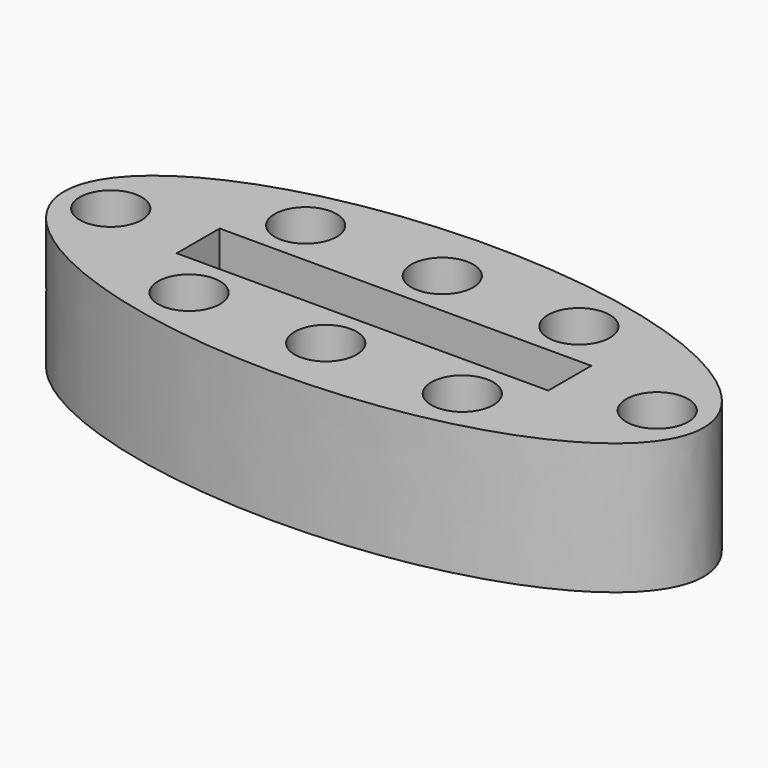
from build123d import *

# Parameters (mm, degrees)
F1_DEPTH = 7.2
F2_W     = 20.4
F2_H     = 2.95
F3_DEPTH = 5.85
F4_W     = 19.15
F4_H     = 1.8
F5_DEPTH = 1.3510001
F6_R     = 1.7
F7_DEPTH = 6.3


# Not quite as in the source:
# - a feature names something its author has since deleted; it is built from what else it names


with BuildPart() as f1:
    # F0 (on Top) → F1 (new body)
    with BuildSketch(Plane.XY):
        with BuildLine():
            add(Edge.make_bspline(
                [(17.5563361044, 0), (17.5563361044, 12.9811752067), (-8.7781680522, 6.4905876034), (-35.1126722087, 0), (-8.7781680522, -6.4905876034), (17.5563361044, -12.9811752067), (17.5563361044, 0)],
                knots=[0, 0, 0, 2.0943951024, 2.0943951024, 4.1887902048, 4.1887902048, 6.2831853072, 6.2831853072, 6.2831853072], degree=2, weights=[1, 0.5, 1, 0.5, 1, 0.5, 1]))
        make_face()
    extrude(amount=F1_DEPTH)

    # F2 (on face) → F3 (cut)
    with BuildSketch(Plane.XY.offset(7.2)):
        Rectangle(F2_W, F2_H)
    extrude(amount=-F3_DEPTH, mode=Mode.SUBTRACT)

    # F4 (on face) → F5 (cut, through all)
    with BuildSketch(Plane.XY.offset(1.35)):
        Rectangle(F4_W, F4_H)
    extrude(amount=-F5_DEPTH, mode=Mode.SUBTRACT)

    # F6 (on face) → F7 (cut)
    with BuildSketch(Plane.XY.offset(7.2)):
        with Locations((-15, 0)):
            Circle(F6_R)
        with Locations((0, 4)):
            Circle(F6_R)
        with Locations((0, -4)):
            Circle(F6_R)
        with Locations((15, 0)):
            Circle(F6_R)
        with Locations((-7.5, 4)):
            Circle(F6_R)
        with Locations((7.5, 4)):
            Circle(F6_R)
        with Locations((7.5, -4)):
            Circle(F6_R)
        with Locations((-7.5, -4)):
            Circle(F6_R)
    extrude(amount=-F7_DEPTH, mode=Mode.SUBTRACT)


solid = f1.part
